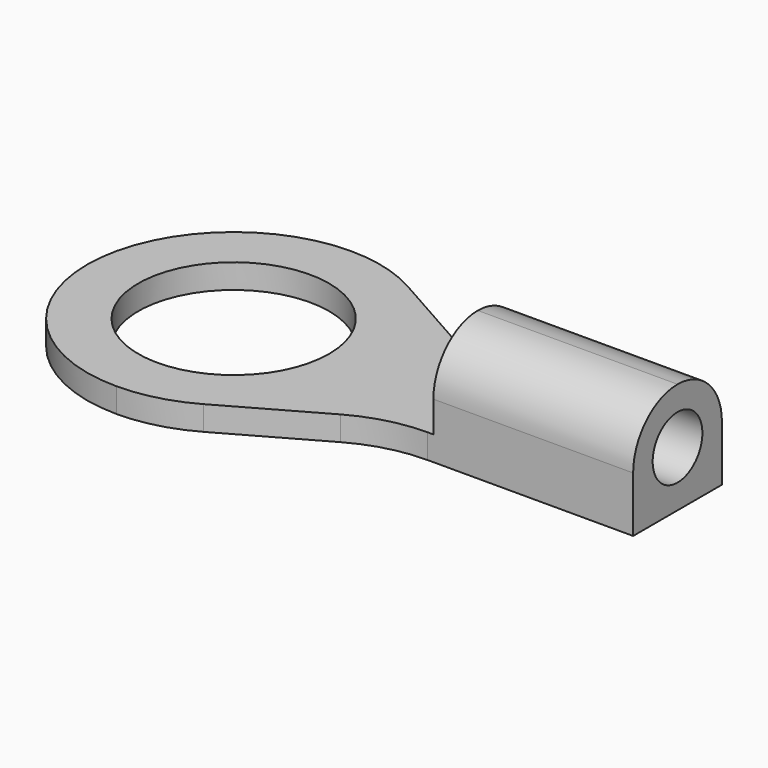
from build123d import *

# Parameters (mm, degrees)
F0_R     = 2.15
F1_DEPTH = 0.55
F2_W     = 4.5
F2_H     = 2.5
F3_DEPTH = 1.95
F4_R     = 1.24999
F5_R     = 0.7
F6_DEPTH = 25


# Not quite as in the source:
# - a fillet or chamfer is up to 0.001 mm smaller than in the source, because OpenCascade refuses the exact size


with BuildPart() as f1:
    # F0 (on Top) → F1 (new body)
    with BuildSketch(Plane.XY):
        with BuildLine():
            Line((8.6667609024, 2.05), (13.3, 2.05))
            Line((13.3, 2.05), (13.3, 4.55))
            Line((13.3, 4.55), (8.6667609024, 4.55))
            ThreePointArc((8.6667609024, 4.55), (7.8284348001, 4.6582591982), (7.0451126442, 4.9759337296))
            Line((7.0451126442, 4.9759337296), (4.9216482582, 6.1740662704))
            ThreePointArc((4.9216482582, 6.1740662704), (4.1383261023, 6.4917408018), (3.3, 6.6))
            ThreePointArc((3.3, 6.6), (0.9665476221, 5.6334523779), (0, 3.3))
            ThreePointArc((0, 3.3), (0.9665476221, 0.9665476221), (3.3, 0))
            ThreePointArc((3.3, 0), (4.1383261023, 0.1082591982), (4.9216482582, 0.4259337296))
            Line((4.9216482582, 0.4259337296), (7.0451126442, 1.6240662704))
            ThreePointArc((7.0451126442, 1.6240662704), (7.8284348001, 1.9417408018), (8.6667609024, 2.05))
        make_face()
        with Locations((3.3, 3.3)):
            Circle(F0_R, mode=Mode.SUBTRACT)
    extrude(amount=F1_DEPTH)

    # F2 (on face) → F3 (join)
    with BuildSketch(Plane.XY.offset(0.55)):
        with Locations((11.05, 3.3)):
            Rectangle(F2_W, F2_H)
    extrude(amount=F3_DEPTH)

    # F4 (radius 1.25 in the source; OpenCascade refuses exactly that, so slightly less here)
    f4_edges = [f1.edges().sort_by_distance(p)[0] for p in [
        (11.05, 4.55, 2.5),
        (11.05, 2.05, 2.5),
    ]]
    fillet(f4_edges, radius=F4_R)

    # F5 (on face) → F6 (cut)
    with BuildSketch(Plane.YZ.offset(13.3)):
        with Locations((3.3, 1.25)):
            Circle(F5_R)
    extrude(amount=-F6_DEPTH, mode=Mode.SUBTRACT)


solid = f1.part
